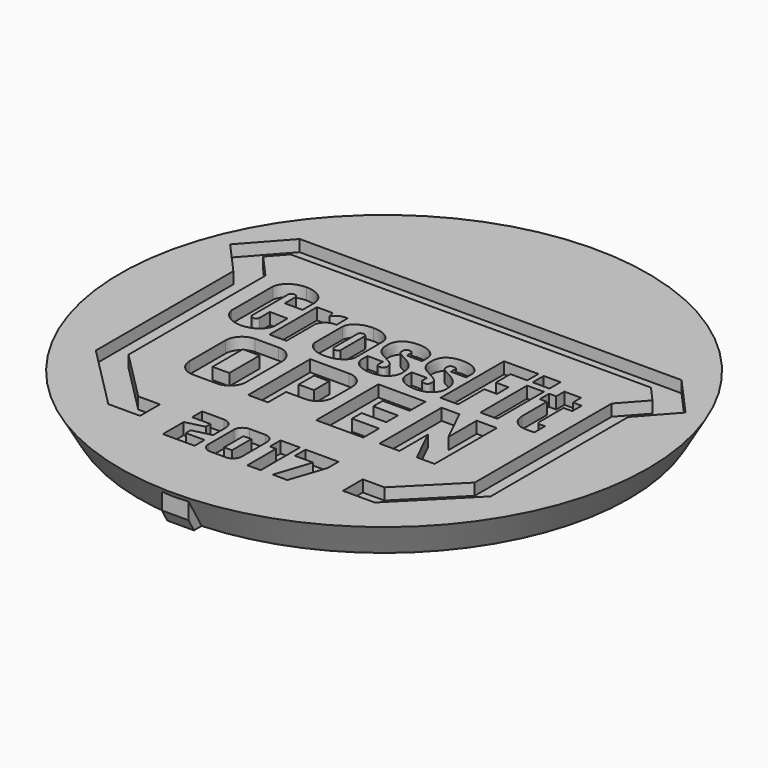
from build123d import *

# Parameters (mm, degrees)
F0_R        = 28.956
F1_DEPTH    = 3.556
F2_W        = 30.4023699468
F2_H        = 2.708328606
F2_W_2      = 1.8437616527
F2_H_2      = 6.3712084666
F2_H_3      = 1.5175901353
F2_W_3      = 1.6611122992
F2_H_4      = 2.0968401222
F2_W_4      = 1.8359664828
F2_H_5      = 4.1484234825
F2_W_5      = 0.8592136437
F2_H_6      = 2.6414245367
F3_DEPTH    = 1.27
F6_DEPTH    = 3.556
F7_T1_DEPTH = 9.4921978168


# Not quite as in the source:
# - a fillet or chamfer that OpenCascade refuses, or shapes differently, is made with other operations: its cross-section is extruded or revolved along the edge and cut away or added


with BuildPart() as f1:
    # F0 (on Top) → F1 (new body)
    with BuildSketch(Plane.XY):
        Circle(F0_R)
    extrude(amount=F1_DEPTH)

    # F2 (on face) → F3 (cut)
    with BuildSketch(Plane.XY.offset(3.556)):
        with Locations((0, 13.1786047998)):
            Rectangle(F2_W, F2_H)
        Polygon((20.8420716974, 14.5327691028), (15.2011849734, 14.5327691028), (15.2011849734, 11.8244404968), (19.6655910583, 11.8244404968), (21.247090707, 10.0590654712), (18.8943144933, 7.4307704384), (18.8943144933, -11.2499324565), (13.4406701729, -16.7418979069), (11.0729235041, -16.7418979069), (11.0729235041, -19.4502265129), (14.5413199249, -19.4502265129), (21.5503721796, -12.3919237413), (21.5503721796, 6.3732514918), (24.849809781, 10.0590654712), align=None)
        Polygon((-15.2011849734, 11.8244404968), (-15.2011849734, 14.5327691028), (-20.8420716974, 14.5327691028), (-24.849809781, 10.0590654712), (-21.5503721796, 6.3732514918), (-21.5503721796, -12.3919237413), (-14.5413199249, -19.4502265129), (-11.0729235041, -19.4502265129), (-11.0729235041, -16.7418979069), (-13.4406701729, -16.7418979069), (-18.8943144933, -11.2499324565), (-18.8943144933, 7.4307704384), (-21.247090707, 10.0590654712), (-19.6655910583, 11.8244404968), align=None)
        with BuildLine():
            ThreePointArc((-15.2091418535, 6.0097032957), (-14.8139919296, 6.2693332665), (-14.4188420058, 6.0097032957))
            Line((-14.4188420058, 6.0097032957), (-14.4188420058, 4.4719388507))
            Line((-14.4188420058, 4.4719388507), (-12.4801692695, 4.4719388507))
            Line((-12.4801692695, 4.4719388507), (-12.4801692695, 6.2930637769))
            add(Edge.make_bspline(
                [(-12.4801692695, 6.2930637769), (-12.5916933403, 6.7707157481), (-12.9251884268, 7.2707731335), (-13.6344023128, 7.7464624472), (-14.2989607428, 7.9362339904), (-14.8139919296, 7.9558056579)],
                knots=[0, 0, 0, 0, 0.3452518733, 0.6338422719, 1, 1, 1, 1], degree=3))
            add(Edge.make_bspline(
                [(-17.1478145898, 6.2930637769), (-17.036290519, 6.7707157481), (-16.7027954325, 7.2707731335), (-15.9935815465, 7.7464624472), (-15.3290231165, 7.9362339904), (-14.8139919296, 7.9558056579)],
                knots=[0, 0, 0, 0, 0.3452518733, 0.6338422719, 1, 1, 1, 1], degree=3))
            Line((-17.1478145898, 6.2930637769), (-17.1478145898, 0.6190669056))
            add(Edge.make_bspline(
                [(-17.1478145898, 0.6190669056), (-17.036290519, 0.1414149345), (-16.7027954325, -0.3586424509), (-15.9935815465, -0.8343317647), (-15.3290231165, -1.0241033079), (-14.8139919296, -1.0436749754)],
                knots=[0, 0, 0, 0, 0.3452518733, 0.6338422719, 1, 1, 1, 1], degree=3))
            add(Edge.make_bspline(
                [(-12.4801692695, 0.6190669056), (-12.5916933403, 0.1414149345), (-12.9251884268, -0.3586424509), (-13.6344023128, -0.8343317647), (-14.2989607428, -1.0241033079), (-14.8139919296, -1.0436749754)],
                knots=[0, 0, 0, 0, 0.3452518733, 0.6338422719, 1, 1, 1, 1], degree=3))
            Line((-12.4801692695, 0.6190669056), (-12.4801692695, 2.4332190197))
            Line((-12.4801692695, 2.4332190197), (-14.4188420058, 2.4332190197))
            Line((-14.4188420058, 2.4332190197), (-14.4188420058, 1.0003426842))
            ThreePointArc((-14.4188420058, 1.0003426842), (-14.8139919296, 0.6797582705), (-15.2091418535, 1.0003426842))
            Line((-15.2091418535, 1.0003426842), (-15.2091418535, 6.0097032957))
        make_face()
        with BuildLine():
            ThreePointArc((-8.498294748, 5.6527445823), (-9.3240459461, 5.52802916), (-9.9700721946, 4.9988136426))
            Line((-9.9700721946, 4.9988136426), (-10.0917066481, 5.6280705877))
            Line((-10.0917066481, 5.6280705877), (-11.8310791474, 5.6280705877))
            Line((-11.8310791474, 5.6280705877), (-11.8310791474, -0.8495571991))
            Line((-11.8310791474, -0.8495571991), (-9.9822352674, -0.8495571991))
            Line((-9.9822352674, -0.8495571991), (-9.9822352674, 3.0987069741))
            ThreePointArc((-9.9822352674, 3.0987069741), (-9.4355214126, 3.8909649876), (-8.498294748, 4.1104529783))
            Line((-8.498294748, 4.1104529783), (-8.498294748, 5.6527445823))
        make_face()
        with BuildLine():
            add(Edge.make_bspline(
                [(-7.8876619975, 4.1982766971), (-7.8356496049, 4.6341372871), (-7.4830251688, 5.0855806361), (-6.6969666534, 5.5265744778), (-6.1764580028, 5.6217318842), (-5.6770178073, 5.6407110794)],
                knots=[0, 0, 0, 0, 0.3397100712, 0.6449265753, 1, 1, 1, 1], degree=3))
            Line((-7.8876619975, 4.1982766971), (-7.8876619975, 0.4633077452))
            add(Edge.make_bspline(
                [(-7.8876619975, 0.4633077452), (-7.8356496049, 0.0274471552), (-7.4830251688, -0.4239961938), (-6.6969666534, -0.8649900355), (-6.1764580028, -0.9601474419), (-5.6770178073, -0.9791266371)],
                knots=[0, 0, 0, 0, 0.3397100712, 0.6449265753, 1, 1, 1, 1], degree=3))
            add(Edge.make_bspline(
                [(-3.4663736171, 0.4633077452), (-3.5183860098, 0.0274471552), (-3.8710104458, -0.4239961938), (-4.6570689612, -0.8649900355), (-5.1775776118, -0.9601474419), (-5.6770178073, -0.9791266371)],
                knots=[0, 0, 0, 0, 0.3397100712, 0.6449265753, 1, 1, 1, 1], degree=3))
            Line((-3.4663736171, 0.4633077452), (-3.4663736171, 4.1982766971))
            add(Edge.make_bspline(
                [(-3.4663736171, 4.1982766971), (-3.5183860098, 4.6341372871), (-3.8710104458, 5.0855806361), (-4.6570689612, 5.5265744778), (-5.1775776118, 5.6217318842), (-5.6770178073, 5.6407110794)],
                knots=[0, 0, 0, 0, 0.3397100712, 0.6449265753, 1, 1, 1, 1], degree=3))
        make_face()
        with BuildLine():
            Line((-6.0537514093, 0.6796154458), (-6.0537514093, 4.0396556988))
            ThreePointArc((-6.0537514093, 4.0396556988), (-5.6770178073, 4.2767262399), (-5.3002842053, 4.0396556988))
            Line((-5.3002842053, 4.0396556988), (-5.3002842053, 0.6796154458))
            ThreePointArc((-5.3002842053, 0.6796154458), (-5.6770178073, 0.4325808427), (-6.0537514093, 0.6796154458))
        make_face(mode=Mode.SUBTRACT)
        with BuildLine():
            add(Edge.make_bspline(
                [(-2.8303159575, 0.3884340668), (-2.8039437057, 0.2035950511), (-2.7084645464, -0.0700189873), (-2.3608920836, -0.4703230086), (-1.9926629718, -0.6996264871), (-1.5028929662, -0.8748491288), (-1.0382407316, -0.9538686812), (-0.6882680471, -0.9546334772), (-0.3368604514, -0.9540527619), (0.2211413136, -0.8513074189), (0.612300795, -0.6901154246), (0.9801185549, -0.3981460143), (1.2267344248, -0.0690546676), (1.3993589582, 0.2977634954), (1.4223729478, 0.7584350911), (1.4049419285, 1.1135593111), (1.3286013981, 1.553696764), (1.1223334914, 1.9521079504), (0.8760135922, 2.2676339155), (0.6015247761, 2.5058684812), (0.2906951276, 2.7053452538), (-0.0001070692, 2.8824823952), (-0.3353974242, 3.0432490404), (-0.5764466432, 3.1792562527), (-0.8154579768, 3.303817088), (-0.9633304165, 3.4276750313), (-1.0959908548, 3.6333141563), (-1.0823984853, 3.8622415727), (-1.0834469924, 4.0754389156), (-0.9485709412, 4.2583690073), (-0.7487440326, 4.3029808765), (-0.5601470729, 4.2949903255), (-0.3773783712, 4.2385764575), (-0.3052749299, 4.1735809243), (-0.2735022713, 4.0681006186)],
                knots=[0, 0, 0, 0, 0.0370250499, 0.0748342879, 0.1100620625, 0.1484988784, 0.1852224027, 0.2162968341, 0.2479903621, 0.2879321478, 0.3230237776, 0.3590762656, 0.3932110531, 0.4269990648, 0.4628119337, 0.4948648069, 0.530192635, 0.5659957163, 0.5996315799, 0.6317213982, 0.6639857771, 0.6953892736, 0.7277821278, 0.7561961656, 0.7835044746, 0.8069782815, 0.8326158776, 0.857980682, 0.8824603672, 0.9067304417, 0.9303429697, 0.953652975, 0.975833924, 1, 1, 1, 1], degree=3))
            Line((-0.2735022713, 4.0681006186), (-0.2735022713, 3.4427449837))
            Line((-0.2735022713, 3.4427449837), (1.3895077923, 3.4427449837))
            Line((1.3895077923, 3.4427449837), (1.3895077923, 4.2547744498))
            add(Edge.make_bspline(
                [(1.3895077923, 4.2547744498), (1.362871865, 4.4414615263), (1.2883734828, 4.7378016949), (0.9605026276, 5.0998324979), (0.5716220009, 5.3815223969), (0.0152610688, 5.5827557819), (-0.3948809767, 5.6297560073), (-0.7047527982, 5.6499225931), (-1.0751777633, 5.6320466323), (-1.6282857111, 5.5504935604), (-2.0336875884, 5.3727640469), (-2.4117723458, 5.0855965451), (-2.6319171142, 4.7457920238), (-2.777638503, 4.3159693257), (-2.7948365878, 3.9652673217), (-2.7867872003, 3.5566089511), (-2.7234512303, 3.1492983197), (-2.4809077804, 2.7167962496), (-2.2560062896, 2.466619706), (-1.9772894721, 2.263975186), (-1.613083499, 2.067015106), (-1.2952433521, 1.9125631017), (-1.0179124703, 1.7567271658), (-0.7490698208, 1.6103729622), (-0.506207899, 1.4077450313), (-0.4071682892, 1.2885965948), (-0.2936071786, 1.0792376552), (-0.3010610885, 0.7910872402), (-0.3213241393, 0.5663172014), (-0.4513056845, 0.4078239751), (-0.6386646385, 0.3709036814), (-0.8427860612, 0.3772912723), (-1.0484772467, 0.4306358217), (-1.1223962588, 0.5223560412), (-1.1560394719, 0.6340462979)],
                knots=[0, 0, 0, 0, 0.0373952344, 0.0734858494, 0.1105806222, 0.1514081281, 0.1855398741, 0.2145930161, 0.246989669, 0.2866513485, 0.3223486125, 0.3583549464, 0.3922575872, 0.4276388924, 0.4592443755, 0.4928782518, 0.5272671439, 0.5643692779, 0.5951310751, 0.6260952205, 0.6604130771, 0.6921960524, 0.7219608284, 0.7518311519, 0.7813056856, 0.8022259164, 0.8274762943, 0.8561110411, 0.8813007038, 0.9041610683, 0.9268832448, 0.9511148768, 0.9744111926, 1, 1, 1, 1], degree=3))
            Line((-1.1560394719, 0.6340462979), (-1.1560394719, 1.2829401795))
            Line((-1.1560394719, 1.2829401795), (-2.8303159575, 1.2829401795))
            Line((-2.8303159575, 1.2829401795), (-2.8303159575, 0.3884340668))
        make_face()
        with BuildLine():
            add(Edge.make_bspline(
                [(1.9797450798, 0.3972758105), (2.0061173315, 0.2124367948), (2.1015964908, -0.0611772436), (2.4491689536, -0.4614812649), (2.8173980654, -0.6907847434), (3.307168071, -0.8660073851), (3.7718203056, -0.9450269375), (4.1217929901, -0.9457917335), (4.4732005858, -0.9452110182), (5.0312023509, -0.8424656752), (5.4223618323, -0.6812736809), (5.7901795921, -0.3893042706), (6.036795462, -0.0602129239), (6.2094199954, 0.3066052391), (6.232433985, 0.7672768348), (6.2150029657, 1.1224010548), (6.1386624353, 1.5625385077), (5.9323945286, 1.9609496941), (5.6860746294, 2.2764756592), (5.4115858133, 2.5147102249), (5.1007561648, 2.7141869975), (4.809953968, 2.8913241389), (4.474663613, 3.0520907841), (4.233614394, 3.1880979964), (3.9946030604, 3.3126588317), (3.8467306207, 3.436516775), (3.7140701824, 3.6421559), (3.7276625519, 3.8710833164), (3.7266140448, 4.0842806593), (3.861490096, 4.267210751), (4.0613170047, 4.3118226202), (4.2499139643, 4.3038320692), (4.4326826661, 4.2474182012), (4.5047861073, 4.182422668), (4.5365587659, 4.0769423623)],
                knots=[0, 0, 0, 0, 0.0370250499, 0.0748342879, 0.1100620625, 0.1484988784, 0.1852224027, 0.2162968341, 0.2479903621, 0.2879321478, 0.3230237776, 0.3590762656, 0.3932110531, 0.4269990648, 0.4628119337, 0.4948648069, 0.530192635, 0.5659957163, 0.5996315799, 0.6317213982, 0.6639857771, 0.6953892736, 0.7277821278, 0.7561961656, 0.7835044746, 0.8069782815, 0.8326158776, 0.857980682, 0.8824603672, 0.9067304417, 0.9303429697, 0.953652975, 0.975833924, 1, 1, 1, 1], degree=3))
            Line((4.5365587659, 4.0769423623), (4.5365587659, 3.4515867274))
            Line((4.5365587659, 3.4515867274), (6.1995688295, 3.4515867274))
            Line((6.1995688295, 3.4515867274), (6.1995688295, 4.2636161935))
            add(Edge.make_bspline(
                [(6.1995688295, 4.2636161935), (6.1729329022, 4.45030327), (6.09843452, 4.7466434386), (5.7705636648, 5.1086742416), (5.3816830381, 5.3903641406), (4.825322106, 5.5915975256), (4.4151800605, 5.638597751), (4.105308239, 5.6587643368), (3.7348832739, 5.640888376), (3.1817753261, 5.5593353041), (2.7763734488, 5.3816057906), (2.3982886914, 5.0944382888), (2.178143923, 4.7546337675), (2.0324225342, 4.3248110694), (2.0152244495, 3.9741090653), (2.0232738369, 3.5654506948), (2.0866098069, 3.1581400634), (2.3291532568, 2.7256379933), (2.5540547477, 2.4754614497), (2.8327715651, 2.2728169297), (3.1969775382, 2.0758568497), (3.5148176851, 1.9214048454), (3.7921485669, 1.7655689095), (4.0609912164, 1.6192147059), (4.3038531382, 1.416586775), (4.402892748, 1.2974383385), (4.5164538586, 1.0880793989), (4.5089999487, 0.7999289839), (4.4887368979, 0.5751589451), (4.3587553528, 0.4166657188), (4.1713963987, 0.3797454251), (3.967274976, 0.386133016), (3.7615837905, 0.4394775654), (3.6876647784, 0.5311977848), (3.6540215653, 0.6428880416)],
                knots=[0, 0, 0, 0, 0.0373952344, 0.0734858494, 0.1105806222, 0.1514081281, 0.1855398741, 0.2145930161, 0.246989669, 0.2866513485, 0.3223486125, 0.3583549464, 0.3922575872, 0.4276388924, 0.4592443755, 0.4928782518, 0.5272671439, 0.5643692779, 0.5951310751, 0.6260952205, 0.6604130771, 0.6921960524, 0.7219608284, 0.7518311519, 0.7813056856, 0.8022259164, 0.8274762943, 0.8561110411, 0.8813007038, 0.9041610683, 0.9268832448, 0.9511148768, 0.9744111926, 1, 1, 1, 1], degree=3))
            Line((3.6540215653, 0.6428880416), (3.6540215653, 1.2917819232))
            Line((3.6540215653, 1.2917819232), (1.9797450798, 1.2917819232))
            Line((1.9797450798, 1.2917819232), (1.9797450798, 0.3972758105))
        make_face()
        Polygon((10.6105204249, 6.2751232445), (10.6105204249, 7.7927133799), (6.8492461505, 7.7927133799), (6.8492461505, -0.854884015), (8.7667587722, -0.854884015), (8.7667587722, 2.7055770889), (10.1574822838, 2.7055770889), (10.1574822838, 4.2872906461), (8.7667587722, 4.2872906461), (8.7667587722, 6.2751232445), align=None)
        with Locations((12.1124403237, 2.3307202183)):
            Rectangle(F2_W_2, F2_H_2)
        with Locations((12.1124403237, 7.0339183122)):
            Rectangle(F2_W_2, F2_H_3)
        with BuildLine():
            Line((16.2016264889, 6.6334225968), (14.3765285406, 6.6334225968))
            Line((14.3765285406, 6.6334225968), (14.3765285406, 5.5163244516))
            Line((14.3765285406, 5.5163244516), (13.5945966262, 5.5163244516))
            Line((13.5945966262, 5.5163244516), (13.5945966262, 4.2304804347))
            Line((13.5945966262, 4.2304804347), (14.3765285406, 4.2304804347))
            Line((14.3765285406, 4.2304804347), (14.3765285406, 0.8540854588))
            ThreePointArc((14.3765285406, 0.8540854588), (14.8770741106, -0.354338445), (16.0854980144, -0.854884015))
            Line((16.0854980144, -0.854884015), (17.0765723828, -0.854884015))
            Line((17.0765723828, -0.854884015), (17.0765723828, 0.6118975844))
            Line((17.0765723828, 0.6118975844), (16.5136363152, 0.6118975844))
            ThreePointArc((16.5136363152, 0.6118975844), (16.2930120512, 0.7032831468), (16.2016264889, 0.9239074107))
            Line((16.2016264889, 0.9239074107), (16.2016264889, 4.2304804347))
            Line((16.2016264889, 4.2304804347), (17.1537883374, 4.2304804347))
            Line((17.1537883374, 4.2304804347), (17.1537883374, 5.5163244516))
            Line((17.1537883374, 5.5163244516), (16.2016264889, 5.5163244516))
            Line((16.2016264889, 5.5163244516), (16.2016264889, 6.6334225968))
        make_face()
        Polygon((9.9929075049, -2.2195314625), (8.0549451523, -2.2195314625), (8.0549451523, -10.6973991598), (10.2406190708, -10.6973991598), (10.2406190708, -6.8355969954), (12.134869583, -10.6973991598), (14.0728319356, -10.6973991598), (14.0728319356, -2.2195314625), (11.887158017, -2.2195314625), (11.887158017, -6.0813336269), align=None)
        Polygon((6.2918351032, -2.2195314625), (1.148215495, -2.2195314625), (1.148215495, -10.6973991598), (6.2918351032, -10.6973991598), (6.2918351032, -8.5553083438), (3.3484606538, -8.5553083438), (3.3484606538, -7.2576974643), (6.0441256501, -7.2576974643), (6.0441256501, -5.6740386746), (3.3484606538, -5.659233158), (3.3484606538, -4.3616222785), (6.2918351032, -4.3616222785), align=None)
        with BuildLine():
            Line((-2.0720108878, -2.2195314625), (-6.28307648, -2.2195314625))
            Line((-6.28307648, -2.2195314625), (-6.28307648, -10.6973991598))
            Line((-6.28307648, -10.6973991598), (-4.1119735688, -10.6973991598))
            Line((-4.1119735688, -10.6973991598), (-4.1119735688, -8.2385173984))
            Line((-4.1119735688, -8.2385173984), (-2.0720108878, -8.2385173984))
            ThreePointArc((-2.0720108878, -8.2385173984), (-0.8289668197, -7.7600961181), (-0.3089004895, -6.5338920205))
            Line((-0.3089004895, -6.5338920205), (-0.3089004895, -3.9241568404))
            ThreePointArc((-0.3089004895, -3.9241568404), (-0.8289668197, -2.6979527428), (-2.0720108878, -2.2195314625))
        make_face()
        with Locations((-3.2959884265, -5.4402171329)):
            Rectangle(F2_W_3, F2_H_4, mode=Mode.SUBTRACT)
        with BuildLine():
            ThreePointArc((-12.3009653762, -2.2195314625), (-13.5702499026, -2.7657857878), (-14.0932183713, -4.0448405081))
            Line((-14.0932183713, -4.0448405081), (-14.0932183713, -8.9475232046))
            ThreePointArc((-14.0932183713, -8.9475232046), (-13.5533866968, -10.1873844568), (-12.3009653762, -10.6973991598))
            Line((-12.3009653762, -10.6973991598), (-9.7364410758, -10.6973991598))
            ThreePointArc((-9.7364410758, -10.6973991598), (-8.443681983, -10.2156752838), (-7.900474593, -8.9475232046))
            Line((-7.900474593, -8.9475232046), (-7.900474593, -4.0448405081))
            ThreePointArc((-7.900474593, -4.0448405081), (-8.4419792148, -2.7535092189), (-9.7364410758, -2.2195314625))
            Line((-9.7364410758, -2.2195314625), (-12.3009653762, -2.2195314625))
        make_face()
        with Locations((-10.9895607457, -6.4509226824)):
            Rectangle(F2_W_4, F2_H_5, mode=Mode.SUBTRACT)
        with BuildLine():
            ThreePointArc((-3.9980014447, -16.5996085636), (-4.3188053633, -15.8251193924), (-5.0932945345, -15.5043154738))
            Line((-5.0932945345, -15.5043154738), (-7.4532657057, -15.5043154738))
            Line((-7.4532657057, -15.5043154738), (-7.4532657057, -16.8733258668))
            Line((-7.4532657057, -16.8733258668), (-5.4378226526, -16.8733258668))
            Line((-5.4378226526, -16.8733258668), (-5.4378226526, -17.5226714457))
            Line((-5.4378226526, -17.5226714457), (-7.4532657057, -18.0188127658))
            Line((-7.4532657057, -18.0188127658), (-7.4532657057, -20.862694544))
            Line((-7.4532657057, -20.862694544), (-3.9980014447, -20.862694544))
            Line((-3.9980014447, -20.862694544), (-3.9980014447, -19.493684151))
            Line((-3.9980014447, -19.493684151), (-6.0480448617, -19.493684151))
            Line((-6.0480448617, -19.493684151), (-6.0480448617, -18.8443385721))
            Line((-6.0480448617, -18.8443385721), (-3.9980014447, -18.3396796855))
            Line((-3.9980014447, -18.3396796855), (-3.9980014447, -16.5996085636))
        make_face()
        with BuildLine():
            Line((-0.556260686, -15.5043154738), (-2.2857946936, -15.5043154738))
            ThreePointArc((-2.2857946936, -15.5043154738), (-2.9607040326, -15.7838720754), (-3.2402606342, -16.4587814144))
            Line((-3.2402606342, -16.4587814144), (-3.2402606342, -19.9082286034))
            ThreePointArc((-3.2402606342, -19.9082286034), (-2.9607040326, -20.5831379424), (-2.2857946936, -20.862694544))
            Line((-2.2857946936, -20.862694544), (-0.556260686, -20.862694544))
            ThreePointArc((-0.556260686, -20.862694544), (0.118648653, -20.5831379424), (0.3982052546, -19.9082286034))
            Line((0.3982052546, -19.9082286034), (0.3982052546, -16.4587814144))
            ThreePointArc((0.3982052546, -16.4587814144), (0.118648653, -15.7838720754), (-0.556260686, -15.5043154738))
        make_face()
        with Locations((-1.418305725, -18.1940381352)):
            Rectangle(F2_W_5, F2_H_6, mode=Mode.SUBTRACT)
        Polygon((3.2210330352, -15.5043154738), (1.1077687483, -15.5043154738), (1.1077687483, -16.9665754709), (1.7710558711, -16.9665754709), (1.7710558711, -20.862694544), (3.2210330352, -20.862694544), align=None)
        Polygon((7.4321370445, -15.5043154738), (3.8380449511, -15.5043154738), (3.8380449511, -16.9665754709), (5.8279069014, -16.9665754709), (4.5321824834, -20.862694544), (6.1364126265, -20.862694544), (7.4321370445, -16.9665754709), align=None)
    extrude(amount=-F3_DEPTH, mode=Mode.SUBTRACT)

    # F4: chamfer of 3.81 x 2.1997045256 on 1 edges, made by hand

    # F4_s1 → F4_t2 (revolve, cut)
    with BuildSketch(Plane.XZ):
        Polygon((28.956, 3.81), (26.7562954744, 0), (28.956, 0), align=None)
    revolve(axis=Axis((0, 0, 0), (0, 0, 1)), mode=Mode.SUBTRACT)

    # F5 (on face) → F6 (join, through all)
    with BuildSketch(Plane.XY.offset(3.556)):
        with BuildLine():
            ThreePointArc((1.4605, -26.7164048342), (0, -26.7562954744), (-1.4605, -26.7164048342))
            Line((-1.4605, -26.7164048342), (-1.4605, -28.4944048342))
            Line((-1.4605, -28.4944048342), (1.4605, -28.4944048342))
            Line((1.4605, -28.4944048342), (1.4605, -26.7164048342))
        make_face()
    extrude(amount=-F6_DEPTH)

    # F7: chamfer of 1.27 x 0.7332348419 on 1 edges, made by hand

    # F7_s2 → F7_t1 (cut)
    with BuildSketch(Plane.YZ.offset(-4.7460989084)):
        Polygon((-27.7611699923, 0), (-28.4944048342, 1.27), (-28.4944048342, 0), align=None)
    extrude(amount=F7_T1_DEPTH, mode=Mode.SUBTRACT)


solid = f1.part
